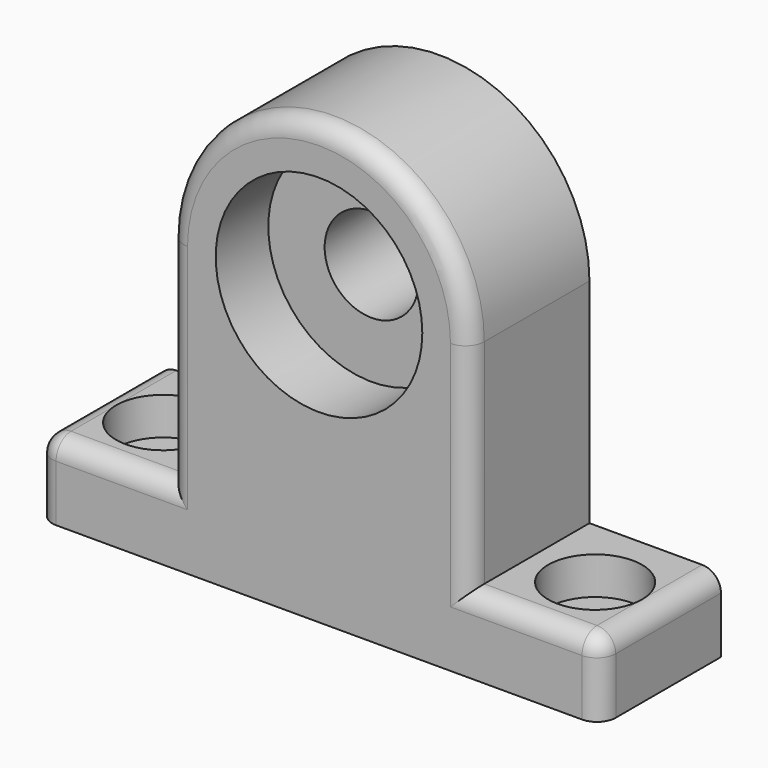
from build123d import *

# Parameters (mm, degrees)
F0_R           = 11
F1_DEPTH       = 8
F3_R           = 11.4612754368
F3_R_2         = 5
F4_DEPTH       = 9
F6_D           = 5
F6_CBORE_D     = 10
F6_CBORE_DEPTH = 4
F7_R           = 1.99999


# Not quite as in the source:
# - a fillet or chamfer is up to 0.001 mm smaller than in the source, because OpenCascade refuses the exact size


with BuildPart() as f1:
    # F0 (on Front) → F1 (new body, symmetric)
    with BuildSketch(Plane.XZ):
        with BuildLine():
            Line((16, 8), (16, 30.7))
            ThreePointArc((16, 30.7), (0, 46.7), (-16, 30.7))
            Line((-16, 30.7), (-16, 8))
            Line((-16, 8), (-30, 8))
            Line((-30, 8), (-30, 0))
            Line((-30, 0), (30, 0))
            Line((30, 0), (30, 8))
            Line((30, 8), (16, 8))
        make_face()
        with Locations((0, 30.7)):
            Circle(F0_R, mode=Mode.SUBTRACT)
    extrude(amount=F1_DEPTH, both=True)

    # F3 (on offset) → F4 (join)
    with BuildSketch(Plane.XZ.offset(1)):
        with Locations((0, 30.7003352791)):
            Circle(F3_R)
        with Locations((0, 30.7003352791)):
            Circle(F3_R_2, mode=Mode.SUBTRACT)
    extrude(amount=-F4_DEPTH)

    # F6 (through all)
    with Locations(Plane.XY.offset(8)):
        with Locations((-23, 0), (23, 0)):
            CounterBoreHole(F6_D / 2, F6_CBORE_D / 2, F6_CBORE_DEPTH)

    # F7 (radius 2 in the source; OpenCascade refuses exactly that, so slightly less here)
    f7_edges = [f1.edges().sort_by_distance(p)[0] for p in [
        (-30, -8, 4),
        (-23, -8, 8),
        (-16, -8, 19.35),
        (23, -8, 8),
        (30, -8, 4),
        (-30, 0, 8),
        (30, 0, 8),
    ]]
    fillet(f7_edges, radius=F7_R)


solid = f1.part
